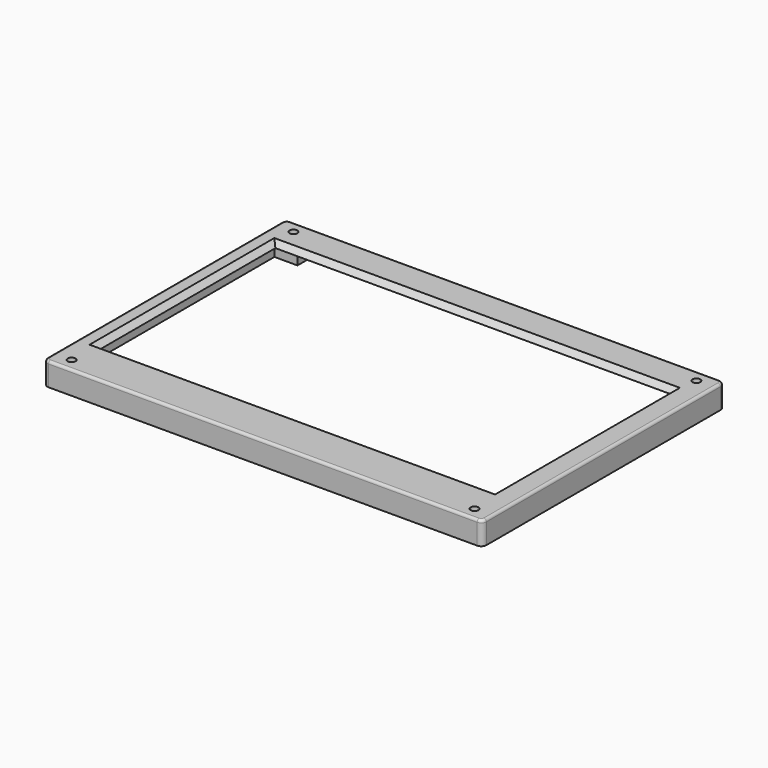
from build123d import *

# Parameters (mm, degrees)
F0_W          = 171
F0_H          = 118
F0_W_2        = 154
F0_H_2        = 86
F1_DEPTH      = 2
F2_SIZE       = 1.99999
F3_R          = 1
F4_W          = 167
F4_H          = 2
F5_DEPTH      = 7
F6_W          = 9
F6_H          = 6
F7_DEPTH      = 7
F8_R          = 1.525
F9_DEPTH      = 9.001
F10_T1_DEPTH  = 14
F10_T4_ANGLE  = 90
F10_T6_ANGLE  = 90
F10_T8_ANGLE  = 90
F10_T10_ANGLE = 90


# Not quite as in the source:
# - a fillet or chamfer that OpenCascade refuses, or shapes differently, is made with other operations: its cross-section is extruded or revolved along the edge and cut away or added
# - a fillet or chamfer is up to 0.001 mm smaller than in the source, because OpenCascade refuses the exact size


with BuildPart() as f1:
    # F0 (on Top) → F1 (new body)
    with BuildSketch(Plane.XY):
        with Locations((1.5, -2.26)):
            Rectangle(F0_W, F0_H)
        with Locations((0, -0.04)):
            Rectangle(F0_W_2, F0_H_2, mode=Mode.SUBTRACT)
    extrude(amount=F1_DEPTH)

    # F2 (size 2 in the source; OpenCascade refuses exactly that, so slightly less here)
    f2_edges = [f1.edges().sort_by_distance(p)[0] for p in [
        (0, 42.96, 2),
        (77, -0.04, 2),
        (-77, -0.04, 2),
        (0, -43.04, 2),
    ]]
    chamfer(f2_edges, length=F2_SIZE)

    # F3
    f3_edges = [f1.edges().sort_by_distance(p)[0] for p in [
        (1.5, -61.26, 2),
        (87, -2.26, 2),
        (1.5, 56.74, 2),
        (-84, -2.26, 2),
    ]]
    fillet(f3_edges, radius=F3_R)

    # F4 (on face) → F5 (join)
    with BuildSketch(Plane(origin=(0, 0, 0), x_dir=(1, 0, 0), z_dir=(0, 0, -1))):
        Polygon((-82, 59.26), (-82, 61.26), (-84, 61.26), (-84, -56.74), (-82, -56.74), (-82, -54.74), align=None)
        Polygon((87, 61.26), (85, 61.26), (85, 59.26), (85, -54.74), (85, -56.74), (87, -56.74), align=None)
        with Locations((1.5, 60.26)):
            Rectangle(F4_W, F4_H)
        with Locations((1.5, -55.74)):
            Rectangle(F4_W, F4_H)
    extrude(amount=F5_DEPTH)

    # F6 (on face) → F7 (join)
    with BuildSketch(Plane(origin=(0, 0, 0), x_dir=(1, 0, 0), z_dir=(0, 0, -1))):
        with Locations((-77.5, 56.26)):
            Rectangle(F6_W, F6_H)
        with Locations((80.5, 56.26)):
            Rectangle(F6_W, F6_H)
        with Locations((80.5, -51.74)):
            Rectangle(F6_W, F6_H)
        with Locations((-77.5, -51.74)):
            Rectangle(F6_W, F6_H)
    extrude(amount=F7_DEPTH)

    # F8 (on face) → F9 (cut, through all)
    with BuildSketch(Plane.XY.offset(2)):
        with Locations((-77, 51.74)):
            Circle(F8_R)
        with Locations((80, 51.74)):
            Circle(F8_R)
        with Locations((80, -56.26)):
            Circle(F8_R)
        with Locations((-77, -56.26)):
            Circle(F8_R)
    extrude(amount=-F9_DEPTH, mode=Mode.SUBTRACT)

    # F10: fillet of radius 2 on 4 edges, made by hand

    # F10_s2 → F10_t1 (cut)
    with BuildSketch(Plane.XY.offset(-12)):
        with BuildLine():
            ThreePointArc((-84, 54.74), (-83.4142135624, 56.1542135624), (-82, 56.74))
            Line((-82, 56.74), (-84, 56.74))
            Line((-84, 56.74), (-84, 54.74))
        make_face()
        with BuildLine():
            ThreePointArc((87, 54.74), (86.4142135624, 56.1542135624), (85, 56.74))
            Line((85, 56.74), (87, 56.74))
            Line((87, 56.74), (87, 54.74))
        make_face()
        with BuildLine():
            ThreePointArc((85, -61.26), (86.4142135624, -60.6742135624), (87, -59.26))
            Line((87, -59.26), (87, -61.26))
            Line((87, -61.26), (85, -61.26))
        make_face()
        with BuildLine():
            ThreePointArc((-82, -61.26), (-83.4142135624, -60.6742135624), (-84, -59.26))
            Line((-84, -59.26), (-84, -61.26))
            Line((-84, -61.26), (-82, -61.26))
        make_face()
    extrude(amount=F10_T1_DEPTH, mode=Mode.SUBTRACT)

    # F10_s3 → F10_t4 (revolve, cut)
    with BuildSketch(Plane.XZ.offset(59.26)):
        with BuildLine():
            ThreePointArc((-83, 2), (-83.7071067812, 1.7071067812), (-84, 1))
            Line((-84, 1), (-84, 2))
            Line((-84, 2), (-83, 2))
        make_face()
    revolve(axis=Axis((-82, -59.26, 2), (0, 0, 1)), revolution_arc=F10_T4_ANGLE, mode=Mode.SUBTRACT)

    # F10_s5 → F10_t6 (revolve, cut)
    with BuildSketch(Plane.YZ.offset(85)):
        with BuildLine():
            ThreePointArc((-60.26, 2), (-60.9671067812, 1.7071067812), (-61.26, 1))
            Line((-61.26, 1), (-61.26, 2))
            Line((-61.26, 2), (-60.26, 2))
        make_face()
    revolve(axis=Axis((85, -59.26, 2), (0, 0, 1)), revolution_arc=F10_T6_ANGLE, mode=Mode.SUBTRACT)

    # F10_s7 → F10_t8 (revolve, cut)
    with BuildSketch(Plane.XZ.offset(-54.74)):
        with BuildLine():
            ThreePointArc((86, 2), (86.7071067812, 1.7071067812), (87, 1))
            Line((87, 1), (87, 2))
            Line((87, 2), (86, 2))
        make_face()
    revolve(axis=Axis((85, 54.74, 2), (0, 0, 1)), revolution_arc=F10_T8_ANGLE, mode=Mode.SUBTRACT)

    # F10_s9 → F10_t10 (revolve, cut)
    with BuildSketch(Plane.YZ.offset(-82)):
        with BuildLine():
            ThreePointArc((55.74, 2), (56.4471067812, 1.7071067812), (56.74, 1))
            Line((56.74, 1), (56.74, 2))
            Line((56.74, 2), (55.74, 2))
        make_face()
    revolve(axis=Axis((-82, 54.74, 2), (0, 0, 1)), revolution_arc=F10_T10_ANGLE, mode=Mode.SUBTRACT)


solid = f1.part
